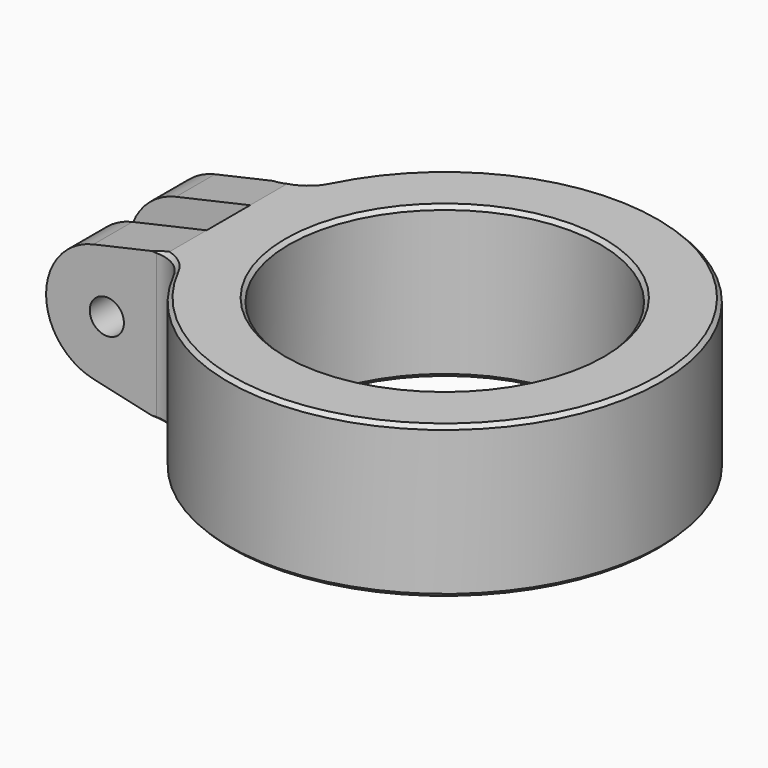
from build123d import *

# Parameters (mm, degrees)
F0_R         = 2.25
F2_DEPTH     = 10
F3_W         = 16
F3_H         = 7.16
F4_DEPTH     = 20.001
F5_R         = 5
F6_T2_ANGLE  = 306.799730078
F6_T4_ANGLE  = 306.799730078
F6_T10_ANGLE = 90.7011440301
F6_T12_ANGLE = 90.7011440301
F6_T14_ANGLE = 90.7011440301
F6_T16_ANGLE = 90.7011440301


# Not quite as in the source:
# - a fillet or chamfer that OpenCascade refuses, or shapes differently, is made with other operations: its cross-section is extruded or revolved along the edge and cut away or added


with BuildPart() as f1:
    # F0 (on Front) → F1 (revolve)
    with BuildSketch(Plane.XZ):
        Polygon((-20.5, 0), (-20.5, 20), (-28.5, 20), (-28.5, 10), (-28.5, 0), align=None)
    revolve(axis=Axis((0, 0, 23.8705657878), (0, 0, -1)))

    # F0 (on Front) → F2 (join, symmetric)
    with BuildSketch(Plane.XZ):
        Polygon((-20.5, 0), (-20.5, 20), (-28.5, 20), (-28.5, 10), (-28.5, 0), align=None)
        with BuildLine():
            Line((-28.5, 10), (-28.5, 20))
            Line((-28.5, 20), (-38.256097561, 17.8048780488))
            ThreePointArc((-38.256097561, 17.8048780488), (-31.5024396196, 16.2469504755), (-28.5, 10))
        make_face()
        with BuildLine():
            Line((-38.256097561, 2.1951219512), (-28.5, 0))
            Line((-28.5, 0), (-28.5, 10))
            ThreePointArc((-28.5, 10), (-31.5024396196, 3.7530495245), (-38.256097561, 2.1951219512))
        make_face()
        with BuildLine():
            ThreePointArc((-38.256097561, 2.1951219512), (-31.5024396196, 3.7530495245), (-28.5, 10))
            ThreePointArc((-28.5, 10), (-31.5024396196, 16.2469504755), (-38.256097561, 17.8048780488))
            ThreePointArc((-38.256097561, 17.8048780488), (-44.5, 10), (-38.256097561, 2.1951219512))
        make_face()
        with Locations((-36.5, 10)):
            Circle(F0_R, mode=Mode.SUBTRACT)
    extrude(amount=F2_DEPTH, both=True)

    # F3 (on face) → F4 (cut, through all)
    with BuildSketch(Plane.XY.offset(20)):
        with Locations((-36.5, 0)):
            Rectangle(F3_W, F3_H)
    extrude(amount=-F4_DEPTH, mode=Mode.SUBTRACT)

    # F5
    f5_edges = [f1.edges().sort_by_distance(p)[0] for p in [
        (-26.688012, 10, 10),
        (-26.688012, -10, 10),
    ]]
    fillet(f5_edges, radius=F5_R)

    # F6: chamfer of 0.5 on 8 edges, made by hand

    # F6_s1 → F6_t2 (revolve, cut)
    with BuildSketch(Plane(origin=(0, 0, 0), x_dir=(0, 0, 1), z_dir=(-0.447761194, -0.8941531821, 0))):
        Polygon((0.5, 28.5), (0, 28), (0, 28.5), align=None)
    revolve(axis=Axis((0, 0, 0), (0, 0, -1)), revolution_arc=F6_T2_ANGLE, mode=Mode.SUBTRACT)

    # F6_s3 → F6_t4 (revolve, cut)
    with BuildSketch(Plane(origin=(0, 0, 0), x_dir=(0, 0, 1), z_dir=(-0.447761194, -0.8941531821, 0))):
        Polygon((20, 28), (19.5, 28.5), (20, 28.5), align=None)
    revolve(axis=Axis((0, 0, 20), (0, 0, -1)), revolution_arc=F6_T4_ANGLE, mode=Mode.SUBTRACT)

    # F6_s5 → F6_t6 (revolve, cut)
    with BuildSketch(Plane.XZ):
        Polygon((-21, 20), (-20.5, 19.5), (-20.5, 20), align=None)
    revolve(axis=Axis((0, 0, 20), (0, 0, -1)), mode=Mode.SUBTRACT)

    # F6_s7 → F6_t8 (revolve, cut)
    with BuildSketch(Plane.XZ):
        Polygon((-20.5, 0.5), (-21, 0), (-20.5, 0), align=None)
    revolve(axis=Axis((0, 0, 0), (0, 0, -1)), mode=Mode.SUBTRACT)

    # F6_s9 → F6_t10 (revolve, cut)
    with BuildSketch(Plane(origin=(-29.7661054166, 15.3642741077, 0), x_dir=(0, 0, 1), z_dir=(-0.8886069942, 0.4586693906, 0))):
        Polygon((20, -5.9099383756), (19.5, -5.4099383756), (20, -5.4099383756), align=None)
    revolve(axis=Axis((-29.9541316015, 15, 20), (0, 0, 1)), revolution_arc=F6_T10_ANGLE, mode=Mode.SUBTRACT)

    # F6_s11 → F6_t12 (revolve, cut)
    with BuildSketch(Plane(origin=(-29.7661054166, -15.3642741077, 0), x_dir=(0, 0, 1), z_dir=(-0.8886069942, -0.4586693906, 0))):
        Polygon((20, 5.9099383756), (19.5, 5.4099383756), (20, 5.4099383756), align=None)
    revolve(axis=Axis((-29.9541316015, -15, 20), (0, 0, -1)), revolution_arc=F6_T12_ANGLE, mode=Mode.SUBTRACT)

    # F6_s13 → F6_t14 (revolve, cut)
    with BuildSketch(Plane(origin=(-29.7661054166, 15.3642741077, 0), x_dir=(0, 0, 1), z_dir=(-0.8886069942, 0.4586693906, 0))):
        Polygon((0.5, -5.4099383756), (0, -5.9099383756), (0, -5.4099383756), align=None)
    revolve(axis=Axis((-29.9541316015, 15, 0), (0, 0, 1)), revolution_arc=F6_T14_ANGLE, mode=Mode.SUBTRACT)

    # F6_s15 → F6_t16 (revolve, cut)
    with BuildSketch(Plane(origin=(-29.7661054166, -15.3642741077, 0), x_dir=(0, 0, 1), z_dir=(-0.8886069942, -0.4586693906, 0))):
        Polygon((0.5, 5.4099383756), (0, 5.9099383756), (0, 5.4099383756), align=None)
    revolve(axis=Axis((-29.9541316015, -15, 0), (0, 0, -1)), revolution_arc=F6_T16_ANGLE, mode=Mode.SUBTRACT)


solid = f1.part
